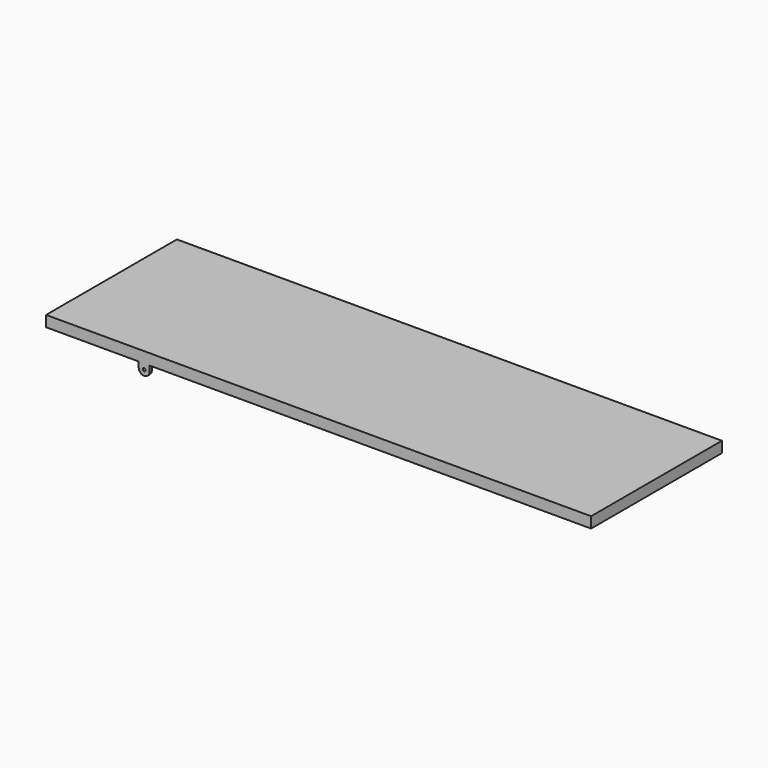
from build123d import *

# Parameters (mm, degrees)
F0_W     = 1270
F0_H     = 381
F1_DEPTH = 25.4
F2_W     = 25.4
F2_H     = 6.35
F3_DEPTH = 25.4
F4_R     = 12.69999
F5_R     = 3.175
F6_DEPTH = 381.001


# Not quite as in the source:
# - a fillet or chamfer is up to 0.001 mm smaller than in the source, because OpenCascade refuses the exact size


with BuildPart() as f1:
    # F0 (on Top) → F1 (new body)
    with BuildSketch(Plane.XY):
        Rectangle(F0_W, F0_H)
    extrude(amount=F1_DEPTH)

    # F2 (on face) → F3 (join)
    with BuildSketch(Plane(origin=(0, 0, 0), x_dir=(1, 0, 0), z_dir=(0, 0, -1))):
        with Locations((-406.4, 187.325)):
            Rectangle(F2_W, F2_H)
        with Locations((-406.4, -187.325)):
            Rectangle(F2_W, F2_H)
    extrude(amount=F3_DEPTH)

    # F4 (radius 12.7 in the source; OpenCascade refuses exactly that, so slightly less here)
    f4_edges = [f1.edges().sort_by_distance(p)[0] for p in [
        (-419.1, -187.325, -25.4),
        (-393.7, -187.325, -25.4),
        (-419.1, 187.325, -25.4),
        (-393.7, 187.325, -25.4),
    ]]
    fillet(f4_edges, radius=F4_R)

    # F5 (on face) → F6 (cut, through all)
    with BuildSketch(Plane(origin=(0, 190.5, 0), x_dir=(-1, 0, 0), z_dir=(0, 1, 0))):
        with Locations((406.4, -12.7)):
            Circle(F5_R)
    extrude(amount=-F6_DEPTH, mode=Mode.SUBTRACT)


solid = f1.part
